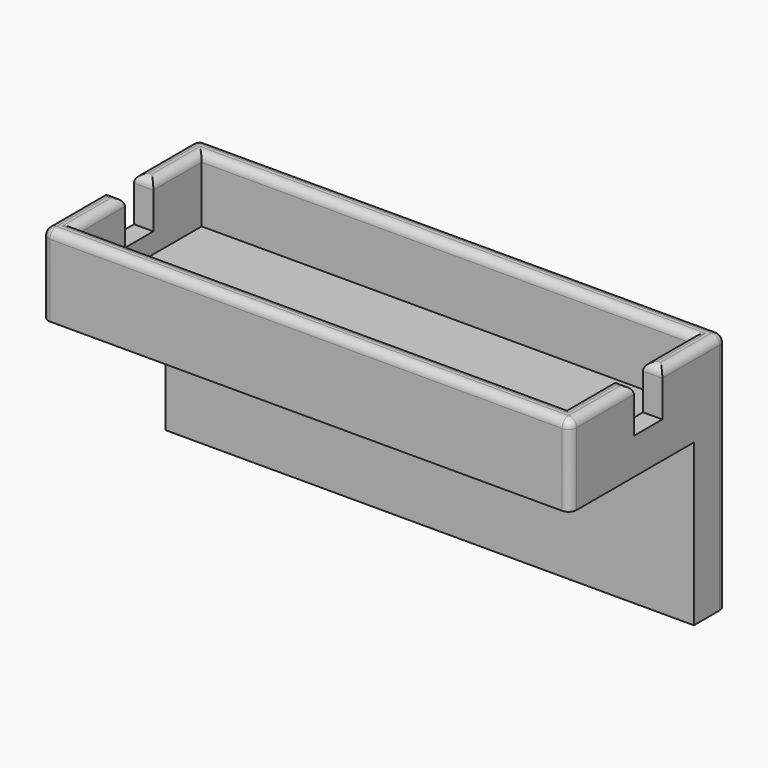
from build123d import *

# Parameters (mm, degrees)
F0_W         = 65.6
F0_H         = 24.2
F0_W_2       = 60.8
F0_H_2       = 19.4
F1_DEPTH     = 10
F2_DEPTH     = 2
F4_DEPTH     = 65.601
F5_W         = 65.6
F5_H         = 20
F6_DEPTH     = 5
F7_R         = 1
F8_R         = 1
F9_T1_DEPTH  = 31.5
F9_T3_DEPTH  = 11.5
F9_S7_W      = 1
F9_S7_H      = 1
F9_T8_DEPTH  = 1
F9_S13_W     = 1
F9_S13_H     = 1
F9_T14_DEPTH = 1
F9_S19_W     = 1
F9_S19_H     = 1
F9_T20_DEPTH = 1
F9_S25_W     = 1
F9_S25_H     = 1
F9_T26_DEPTH = 1


# Not quite as in the source:
# - a fillet or chamfer that OpenCascade refuses, or shapes differently, is made with other operations: its cross-section is extruded or revolved along the edge and cut away or added


with BuildPart() as f1:
    # F0 (on Top) → F1 (new body)
    with BuildSketch(Plane.XY):
        Rectangle(F0_W, F0_H)
        Rectangle(F0_W_2, F0_H_2, mode=Mode.SUBTRACT)
    extrude(amount=F1_DEPTH)

    # F0 (on Top) → F2 (join)
    with BuildSketch(Plane.XY):
        Rectangle(F0_W_2, F0_H_2)
    extrude(amount=F2_DEPTH)

    # F3 (on face) → F4 (cut, through all)
    with BuildSketch(Plane.YZ.offset(32.8)):
        Polygon((2.2, 10), (0, 10), (-2.2, 10), (-2.2, 4.5), (0, 4.5), (2.2, 4.5), align=None)
    extrude(amount=-F4_DEPTH, mode=Mode.SUBTRACT)

    # F5 (on face) → F6 (join)
    with BuildSketch(Plane(origin=(0, 12.1, 0), x_dir=(-1, 0, 0), z_dir=(0, 1, 0))):
        with Locations((0, -10)):
            Rectangle(F5_W, F5_H)
    extrude(amount=-F6_DEPTH)

    # F7
    f7_edges = [f1.edges().sort_by_distance(p)[0] for p in [
        (0, -9.7, 10),
        (0, -12.1, 10),
        (-32.8, -7.15, 10),
        (32.8, -7.15, 10),
        (30.4, -5.95, 10),
        (-31.6, -2.2, 10),
        (31.6, -2.2, 10),
        (-30.4, -5.95, 10),
    ]]
    fillet(f7_edges, radius=F7_R)

    # F8
    f8_edges = [f1.edges().sort_by_distance(p)[0] for p in [
        (-31.6, 2.2, 10),
        (31.6, 2.2, 10),
        (32.8, 7.15, 10),
        (-32.8, 7.15, 10),
        (-30.4, 5.95, 10),
        (30.4, 5.95, 10),
        (0, 9.7, 10),
        (0, 12.1, 10),
    ]]
    fillet(f8_edges, radius=F8_R)

    # F9: fillet of radius 1 on 4 edges, made by hand

    # F9_s2 → F9_t1 (cut)
    with BuildSketch(Plane.XY.offset(-22.5)):
        with BuildLine():
            ThreePointArc((31.8, 12.1), (32.5071067812, 11.8071067812), (32.8, 11.1))
            Line((32.8, 11.1), (32.8, 12.1))
            Line((32.8, 12.1), (31.8, 12.1))
        make_face()
        with BuildLine():
            ThreePointArc((-32.8, 11.1), (-32.5071067812, 11.8071067812), (-31.8, 12.1))
            Line((-31.8, 12.1), (-32.8, 12.1))
            Line((-32.8, 12.1), (-32.8, 11.1))
        make_face()
    extrude(amount=F9_T1_DEPTH, mode=Mode.SUBTRACT)

    # F9_s4 → F9_t3 (cut)
    with BuildSketch(Plane.XY.offset(-2.5)):
        with BuildLine():
            ThreePointArc((31.8, -12.1), (32.5071067812, -11.8071067812), (32.8, -11.1))
            Line((32.8, -11.1), (32.8, -12.1))
            Line((32.8, -12.1), (31.8, -12.1))
        make_face()
        with BuildLine():
            ThreePointArc((-32.8, -11.1), (-32.5071067812, -11.8071067812), (-31.8, -12.1))
            Line((-31.8, -12.1), (-32.8, -12.1))
            Line((-32.8, -12.1), (-32.8, -11.1))
        make_face()
    extrude(amount=F9_T3_DEPTH, mode=Mode.SUBTRACT)


with BuildPart() as f9_tool6:
    # F9_s7 → F9_t8 (new body)
    with BuildSketch(Plane.YZ.offset(-31.8)):
        with Locations((-11.6, 9.5)):
            Rectangle(F9_S7_W, F9_S7_H)
    extrude(amount=-F9_T8_DEPTH)

    # F9_s9 → F9_t10 (revolve, cut)
    with BuildSketch(Plane(origin=(-31.8, -11.1, 9), x_dir=(0, 0.7071067812, -0.7071067812), z_dir=(0, 0.7071067812, 0.7071067812))):
        with BuildLine():
            ThreePointArc((0, -1), (1, 0), (0, 1))
            Line((0, 1), (0, -1))
        make_face()
    revolve(axis=Axis((-31.8, -11.1, 9), (-1, 0, 0)), mode=Mode.SUBTRACT)


with BuildPart() as f1_1:
    add(f1.part)

    # F9_t5: cut F9_tool6
    add(f9_tool6.part, mode=Mode.SUBTRACT)


with BuildPart() as f9_tool12:
    # F9_s13 → F9_t14 (new body)
    with BuildSketch(Plane.YZ.offset(-31.8)):
        with Locations((11.6, 9.5)):
            Rectangle(F9_S13_W, F9_S13_H)
    extrude(amount=-F9_T14_DEPTH)

    # F9_s15 → F9_t16 (revolve, cut)
    with BuildSketch(Plane(origin=(-31.8, 11.1, 9), x_dir=(0, -0.7071067812, -0.7071067812), z_dir=(0, 0.7071067812, -0.7071067812))):
        with BuildLine():
            ThreePointArc((0, -1), (1, 0), (0, 1))
            Line((0, 1), (0, -1))
        make_face()
    revolve(axis=Axis((-31.8, 11.1, 9), (-1, 0, 0)), mode=Mode.SUBTRACT)


with BuildPart() as f1_2:
    add(f1_1.part)

    # F9_t11: cut F9_tool12
    add(f9_tool12.part, mode=Mode.SUBTRACT)


with BuildPart() as f9_tool18:
    # F9_s19 → F9_t20 (new body)
    with BuildSketch(Plane.XZ.offset(11.1)):
        with Locations((32.3, 9.5)):
            Rectangle(F9_S19_W, F9_S19_H)
    extrude(amount=F9_T20_DEPTH)

    # F9_s21 → F9_t22 (revolve, cut)
    with BuildSketch(Plane(origin=(31.8, -11.1, 9), x_dir=(-0.7071067812, 0, -0.7071067812), z_dir=(-0.7071067812, 0, 0.7071067812))):
        with BuildLine():
            ThreePointArc((0, -1), (1, 0), (0, 1))
            Line((0, 1), (0, -1))
        make_face()
    revolve(axis=Axis((31.8, -11.1, 9), (0, -1, 0)), mode=Mode.SUBTRACT)


with BuildPart() as f1_3:
    add(f1_2.part)

    # F9_t17: cut F9_tool18
    add(f9_tool18.part, mode=Mode.SUBTRACT)


with BuildPart() as f9_tool24:
    # F9_s25 → F9_t26 (new body)
    with BuildSketch(Plane.XZ.offset(-11.1)):
        with Locations((32.3, 9.5)):
            Rectangle(F9_S25_W, F9_S25_H)
    extrude(amount=-F9_T26_DEPTH)

    # F9_s27 → F9_t28 (revolve, cut)
    with BuildSketch(Plane(origin=(31.8, 11.1, 9), x_dir=(-0.7071067812, 0, -0.7071067812), z_dir=(0.7071067812, 0, -0.7071067812))):
        with BuildLine():
            ThreePointArc((0, -1), (1, 0), (0, 1))
            Line((0, 1), (0, -1))
        make_face()
    revolve(axis=Axis((31.8, 11.1, 9), (0, 1, 0)), mode=Mode.SUBTRACT)


with BuildPart() as f1_4:
    add(f1_3.part)

    # F9_t23: cut F9_tool24
    add(f9_tool24.part, mode=Mode.SUBTRACT)


solid = f1_4.part
